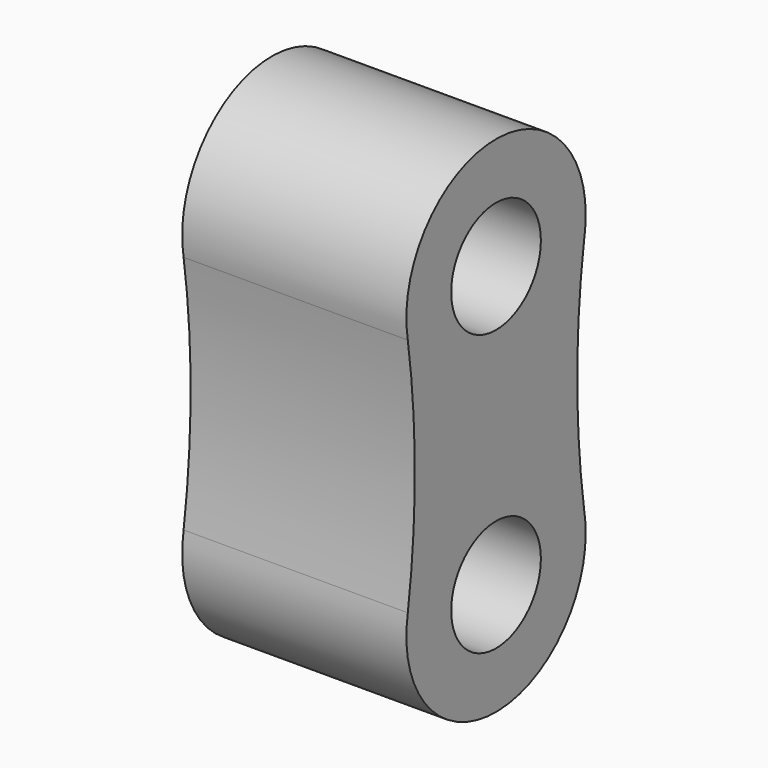
from build123d import *

# Parameters (mm, degrees)
F0_R     = 6.35
F1_DEPTH = 25.4


# Not quite as in the source:
# - a feature names something its author has since deleted; it is built from what else it names


with BuildPart() as f1:
    # F0 (on Right) → F1 (new body)
    with BuildSketch(Plane.YZ):
        with BuildLine():
            ThreePointArc((12.4942827194, 13.5984018078), (12.6484661231, 14.7320631111), (12.7, 15.875))
            ThreePointArc((12.7, 15.875), (-1.1429368889, 28.5234661231), (-12.4942827194, 13.5984018078))
            ThreePointArc((-12.4942827194, 13.5984018078), (0, 3.175), (12.4942827194, 13.5984018078))
        make_face()
        with Locations((0, 15.875)):
            Circle(F0_R, mode=Mode.SUBTRACT)
        with BuildLine():
            ThreePointArc((12.4942827194, -13.5984018078), (0, -3.175), (-12.4942827194, -13.5984018078))
            ThreePointArc((-12.4942827194, -13.5984018078), (-1.1429368889, -28.5234661231), (12.7, -15.875))
            ThreePointArc((12.7, -15.875), (12.6484661231, -14.7320631111), (12.4942827194, -13.5984018078))
        make_face()
        with Locations((0, -15.875)):
            Circle(F0_R, mode=Mode.SUBTRACT)
        with BuildLine():
            ThreePointArc((12.4942827194, 13.5984018078), (0, 3.175), (-12.4942827194, 13.5984018078))
            ThreePointArc((-12.4942827194, 13.5984018078), (-11.5006568446, 0), (-12.4942827194, -13.5984018078))
            ThreePointArc((-12.4942827194, -13.5984018078), (0, -3.175), (12.4942827194, -13.5984018078))
            ThreePointArc((12.4942827194, -13.5984018078), (11.5006568446, 0), (12.4942827194, 13.5984018078))
        make_face()
    extrude(amount=F1_DEPTH)


solid = f1.part
